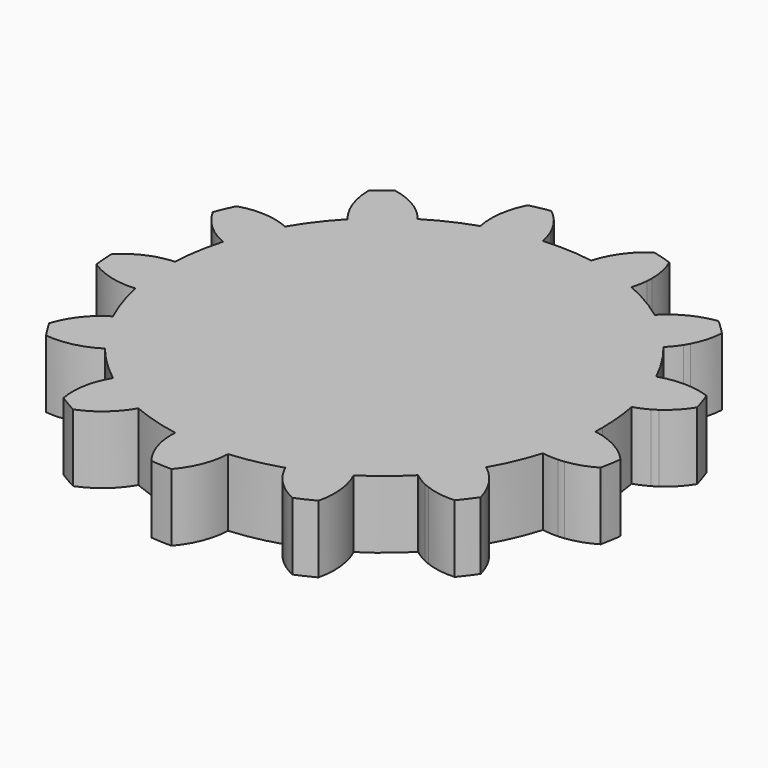
from build123d import *

# Parameters (mm, degrees)
F1_DEPTH = 6.35
F2_COUNT = 13


with BuildPart() as f1:
    # F0 (on Top) → F1 (new body)
    with BuildSketch(Plane.XY):
        with BuildLine():
            ThreePointArc((7.9296197565, 23.5951858335), (6.9911317973, 23.8900761864), (6.0417249702, 24.1476546146))
            ThreePointArc((6.0417249702, 24.1476546146), (4.3226425573, 22.4330749308), (3.2648662162, 20.2476374354))
            ThreePointArc((3.2648662162, 20.2476374354), (5.7837443287, 19.6767495961), (8.2108987358, 18.7938105523))
            ThreePointArc((8.2108987358, 18.7938105523), (8.3954934616, 19.5156536929), (8.4994507341, 20.2534379554))
            ThreePointArc((8.4994507341, 20.2534379554), (8.5176465567, 20.5391701676), (8.5237154667, 20.8254168329))
            ThreePointArc((8.5237154667, 20.8254168329), (8.373521449, 22.2418004346), (7.9296197565, 23.5951858335))
        make_face()
        with BuildLine():
            ThreePointArc((4.0264902572, 14.4598933509), (-1.7431476836, 15.057566034), (-4.9211585336, 19.9100068261))
            ThreePointArc((-4.9211585336, 19.9100068261), (-12.6431262329, -16.1486077476), (20.5091729021, 0))
            ThreePointArc((20.5091729021, 0), (19.2415803806, 7.0984334598), (15.5954927821, 13.3194135761))
            ThreePointArc((15.5954927821, 13.3194135761), (9.5256046991, 10.9946956396), (4.0264902572, 14.4598933509))
        make_face()
        with BuildLine():
            ThreePointArc((3.2648662162, 20.2476374354), (-0.8451772993, 20.4917507417), (-4.9211585336, 19.9100068261))
            ThreePointArc((-4.9211585336, 19.9100068261), (-1.7431476836, 15.057566034), (4.0264902572, 14.4598933509))
            ThreePointArc((4.0264902572, 14.4598933509), (3.0384725246, 17.2738616412), (3.2648662162, 20.2476374354))
        make_face()
        with BuildLine():
            ThreePointArc((4.0264902572, 14.4598933509), (9.5256046991, 10.9946956396), (15.5954927821, 13.3194135761))
            ThreePointArc((15.5954927821, 13.3194135761), (12.2138579016, 16.4756744411), (8.2108987358, 18.7938105523))
            ThreePointArc((8.2108987358, 18.7938105523), (6.6287005247, 16.1344397874), (4.0264902572, 14.4598933509))
        make_face()
        with BuildLine():
            ThreePointArc((8.2108987358, 18.7938105523), (5.7837443287, 19.6767495961), (3.2648662162, 20.2476374354))
            ThreePointArc((3.2648662162, 20.2476374354), (3.0384725246, 17.2738616412), (4.0264902572, 14.4598933509))
            ThreePointArc((4.0264902572, 14.4598933509), (6.6287005247, 16.1344397874), (8.2108987358, 18.7938105523))
        make_face()
    extrude(amount=F1_DEPTH)

    # F2: F1 ×13 about axis
    f2_axis = Axis((0, 0, 6.35), (0, 0, 1))


with BuildPart() as f1_1:
    add(f1.part)
    for i in range(1, F2_COUNT):
        add(f1.part.rotate(f2_axis, i * 360 / F2_COUNT))


solid = f1_1.part
